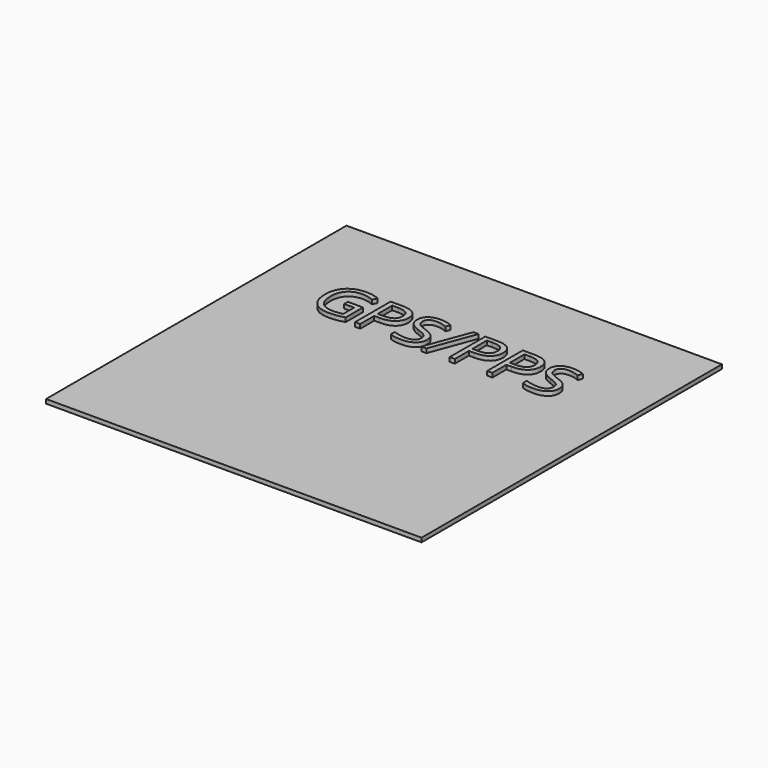
from build123d import *

# Parameters (mm, degrees)
F0_W         = 114.3
F0_H         = 114.3
F1_DEPTH     = 1.27
F2_TEXT_SIZE = 18.9743988795
F3_DEPTH     = 1.27


# Not quite as in the source:
# - Text() gives the source's letters only with a copy of the font that has no kerning and outlines rounded to 1/6400 em; it was checked with that copy


with BuildPart() as f1:
    # F0 (on Top) → F1 (new body)
    with BuildSketch(Plane.XY):
        with Locations((2.4647638202, 10.536187025)):
            Rectangle(F0_W, F0_H)
    extrude(amount=F1_DEPTH)

    # F2 (on face) → F3 (join)
    with BuildSketch(Plane.XY.offset(1.27)):
        with Locations((-36.2027871711, 28.2559511226)):
            Text('GPS/PPS', F2_TEXT_SIZE, font='Open Sans', text_align=(TextAlign.LEFT, TextAlign.BOTTOM))
    extrude(amount=F3_DEPTH)


solid = f1.part
